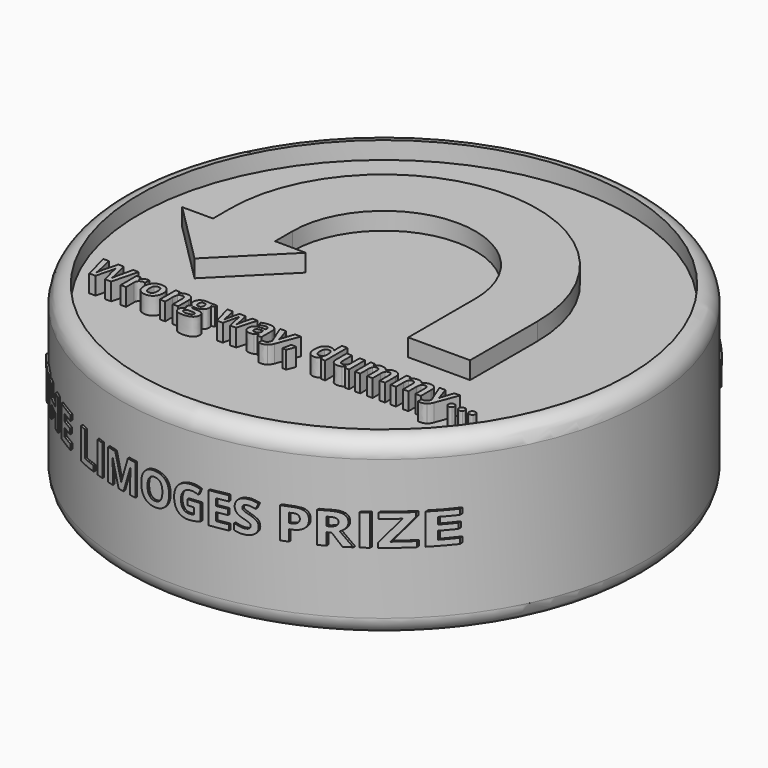
from build123d import *

# Parameters (mm, degrees)
F0_R         = 38.1
F1_DEPTH     = 25.4
F2_R         = 2.54
F3_R         = 35.56
F4_DEPTH     = 2.54
F5_DEPTH     = 2.54
F6_DEPTH     = 2.54
F8_TEXT_SIZE = 6.3120904723
F9_DEPTH     = 15.24
F10_R        = 50.5261755915
F10_R_2      = 38.354
F11_DEPTH    = 25.4
F13_COUNT    = 2
F13_ANGLE    = 180


# Not quite as in the source:
# - Text() gives the source's letters only with a copy of the font that has no kerning and outlines rounded to 1/6400 em; it was checked with that copy


with BuildPart() as f1:
    # F0 (on Top) → F1 (new body)
    with BuildSketch(Plane.XY):
        Circle(F0_R)
    extrude(amount=F1_DEPTH)

    # F2
    f2_edges = [f1.edges().sort_by_distance(p)[0] for p in [
        (-38.1, 0, 25.4),
        (-38.1, 0, 0),
    ]]
    fillet(f2_edges, radius=F2_R)

    # F3 (on face) → F4 (cut)
    with BuildSketch(Plane.XY.offset(25.4)):
        Circle(F3_R)
        with BuildLine():
            Line((-12.6157349895, -15.8383565248), (-11.6065968712, -15.8383565248))
            Line((-11.6065968712, -15.8383565248), (-11.6065968712, -16.2398593857))
            Line((-11.6065968712, -16.2398593857), (-12.0594258709, -16.3557571187))
            add(Edge.make_bspline(
                [(-12.0594258709, -16.3557571187), (-11.9352497284, -16.550299742), (-11.9352497284, -16.7903736176)],
                knots=[0, 0, 0, 1, 1, 1], degree=2))
            add(Edge.make_bspline(
                [(-11.9352497284, -16.7903736176), (-11.9352497284, -17.2564480726), (-12.2601773014, -17.516390131)],
                knots=[0, 0, 0, 1, 1, 1], degree=2))
            add(Edge.make_bspline(
                [(-12.2601773014, -17.516390131), (-12.5851048743, -17.7763321893), (-13.1612821757, -17.7763321893)],
                knots=[0, 0, 0, 1, 1, 1], degree=2))
            Line((-13.1612821757, -17.7763321893), (-13.3036708191, -17.7680537798))
            Line((-13.3036708191, -17.7680537798), (-13.4203963931, -17.7556361656))
            add(Edge.make_bspline(
                [(-13.4203963931, -17.7556361656), (-13.5420890128, -17.848354352), (-13.5420890128, -17.9625964031)],
                knots=[0, 0, 0, 1, 1, 1], degree=2))
            add(Edge.make_bspline(
                [(-13.5420890128, -17.9625964031), (-13.5420890128, -18.1331316389), (-13.1074725139, -18.1331316389)],
                knots=[0, 0, 0, 1, 1, 1], degree=2))
            Line((-13.1074725139, -18.1331316389), (-12.6157349895, -18.1331316389))
            add(Edge.make_bspline(
                [(-12.6157349895, -18.1331316389), (-12.1397264431, -18.1331316389), (-11.8901323966, -18.3376083536)],
                knots=[0, 0, 0, 1, 1, 1], degree=2))
            add(Edge.make_bspline(
                [(-11.8901323966, -18.3376083536), (-11.6405383501, -18.5420850683), (-11.6405383501, -18.9377930425)],
                knots=[0, 0, 0, 1, 1, 1], degree=2))
            add(Edge.make_bspline(
                [(-11.6405383501, -18.9377930425), (-11.6405383501, -19.445259545), (-12.0635650757, -19.7246558657)],
                knots=[0, 0, 0, 1, 1, 1], degree=2))
            add(Edge.make_bspline(
                [(-12.0635650757, -19.7246558657), (-12.4865918013, -20.0040521864), (-13.2780077497, -20.0040521864)],
                knots=[0, 0, 0, 1, 1, 1], degree=2))
            add(Edge.make_bspline(
                [(-13.2780077497, -20.0040521864), (-13.8831594843, -20.0040521864), (-14.2027060911, -19.7929527441)],
                knots=[0, 0, 0, 1, 1, 1], degree=2))
            add(Edge.make_bspline(
                [(-14.2027060911, -19.7929527441), (-14.5222526979, -19.5818533018), (-14.5222526979, -19.2018743057)],
                knots=[0, 0, 0, 1, 1, 1], degree=2))
            add(Edge.make_bspline(
                [(-14.5222526979, -19.2018743057), (-14.5222526979, -18.9402765654), (-14.3591680307, -18.7643603635)],
                knots=[0, 0, 0, 1, 1, 1], degree=2))
            add(Edge.make_bspline(
                [(-14.3591680307, -18.7643603635), (-14.1960833635, -18.5884441615), (-13.8806759615, -18.5131106351)],
                knots=[0, 0, 0, 1, 1, 1], degree=2))
            add(Edge.make_bspline(
                [(-13.8806759615, -18.5131106351), (-14.0023685812, -18.4617844961), (-14.0930171652, -18.3442310812)],
                knots=[0, 0, 0, 1, 1, 1], degree=2))
            add(Edge.make_bspline(
                [(-14.0930171652, -18.3442310812), (-14.1836657493, -18.2266776663), (-14.1836657493, -18.0942231142)],
                knots=[0, 0, 0, 1, 1, 1], degree=2))
            add(Edge.make_bspline(
                [(-14.1836657493, -18.0942231142), (-14.1836657493, -17.9286549242), (-14.0880501195, -17.8189659983)],
                knots=[0, 0, 0, 1, 1, 1], degree=2))
            add(Edge.make_bspline(
                [(-14.0880501195, -17.8189659983), (-13.9924344898, -17.7092770724), (-13.8111373216, -17.6024855898)],
                knots=[0, 0, 0, 1, 1, 1], degree=2))
            add(Edge.make_bspline(
                [(-13.8111373216, -17.6024855898), (-14.038793583, -17.5048003577), (-14.172075976, -17.2874921082)],
                knots=[0, 0, 0, 1, 1, 1], degree=2))
            add(Edge.make_bspline(
                [(-14.172075976, -17.2874921082), (-14.3053583689, -17.0701838588), (-14.3053583689, -16.7746446395)],
                knots=[0, 0, 0, 1, 1, 1], degree=2))
            add(Edge.make_bspline(
                [(-14.3053583689, -16.7746446395), (-14.3053583689, -16.301947457), (-13.9974015355, -16.04324716)],
                knots=[0, 0, 0, 1, 1, 1], degree=2))
            add(Edge.make_bspline(
                [(-13.9974015355, -16.04324716), (-13.689444702, -15.7845468631), (-13.1174066053, -15.7845468631)],
                knots=[0, 0, 0, 1, 1, 1], degree=2))
            add(Edge.make_bspline(
                [(-13.1174066053, -15.7845468631), (-12.9957139857, -15.7845468631), (-12.8289040342, -15.8064846482)],
                knots=[0, 0, 0, 1, 1, 1], degree=2))
            add(Edge.make_bspline(
                [(-12.8289040342, -15.8064846482), (-12.6620940827, -15.8284224334), (-12.6157349895, -15.8383565248)],
                knots=[0, 0, 0, 1, 1, 1], degree=2))
        make_face(mode=Mode.SUBTRACT)
        with BuildLine():
            Line((-1.2834202216, -18.7101367812), (-2.4324634606, -15.8383565248))
            Line((-2.4324634606, -15.8383565248), (-1.5681975085, -15.8383565248))
            Line((-1.5681975085, -15.8383565248), (-1.0226503223, -17.465891833))
            add(Edge.make_bspline(
                [(-1.0226503223, -17.465891833), (-0.9522838415, -17.6778191163), (-0.9266207721, -17.9675634488)],
                knots=[0, 0, 0, 1, 1, 1], degree=2))
            Line((-0.9266207721, -17.9675634488), (-0.910891794, -17.9675634488))
            add(Edge.make_bspline(
                [(-0.910891794, -17.9675634488), (-0.8827452017, -17.7009986629), (-0.7999611067, -17.465891833)],
                knots=[0, 0, 0, 1, 1, 1], degree=2))
            Line((-0.7999611067, -17.465891833), (-0.2643480119, -15.8383565248))
            Line((-0.2643480119, -15.8383565248), (0.5817054393, -15.8383565248))
            Line((0.5817054393, -15.8383565248), (-0.6418434852, -19.1008777097))
            add(Edge.make_bspline(
                [(-0.6418434852, -19.1008777097), (-0.810723039, -19.5537067095), (-1.1224051568, -19.778879448)],
                knots=[0, 0, 0, 1, 1, 1], degree=2))
            add(Edge.make_bspline(
                [(-1.1224051568, -19.778879448), (-1.4340872746, -20.0040521864), (-1.8504912725, -20.0040521864)],
                knots=[0, 0, 0, 1, 1, 1], degree=2))
            add(Edge.make_bspline(
                [(-1.8504912725, -20.0040521864), (-2.0549679873, -20.0040521864), (-2.2511662925, -19.9593487751)],
                knots=[0, 0, 0, 1, 1, 1], degree=2))
            Line((-2.2511662925, -19.9593487751), (-2.2511662925, -19.3335010167))
            add(Edge.make_bspline(
                [(-2.2511662925, -19.3335010167), (-2.108777649, -19.3674424957), (-1.9407259361, -19.3674424957)],
                knots=[0, 0, 0, 1, 1, 1], degree=2))
            add(Edge.make_bspline(
                [(-1.9407259361, -19.3674424957), (-1.7312821757, -19.3674424957), (-1.5748202361, -19.2391271484)],
                knots=[0, 0, 0, 1, 1, 1], degree=2))
            add(Edge.make_bspline(
                [(-1.5748202361, -19.2391271484), (-1.4183582965, -19.1108118011), (-1.3306071558, -18.8525254247)],
                knots=[0, 0, 0, 1, 1, 1], degree=2))
            Line((-1.3306071558, -18.8525254247), (-1.2834202216, -18.7101367812))
        make_face(mode=Mode.SUBTRACT)
        with BuildLine():
            Line((-23.7063201999, -14.9484275033), (-24.669099225, -18.730832805))
            Line((-24.669099225, -18.730832805), (-25.5822077931, -18.730832805))
            Line((-25.5822077931, -18.730832805), (-26.0946413413, -16.7440145244))
            add(Edge.make_bspline(
                [(-26.0946413413, -16.7440145244), (-26.1227879337, -16.6380508828), (-26.1914987325, -16.3056727412)],
                knots=[0, 0, 0, 1, 1, 1], degree=2))
            add(Edge.make_bspline(
                [(-26.1914987325, -16.3056727412), (-26.2602095314, -15.9732945997), (-26.2701436228, -15.8590525486)],
                knots=[0, 0, 0, 1, 1, 1], degree=2))
            add(Edge.make_bspline(
                [(-26.2701436228, -15.8590525486), (-26.2858726009, -15.9989576692), (-26.3479606721, -16.3081562641)],
                knots=[0, 0, 0, 1, 1, 1], degree=2))
            add(Edge.make_bspline(
                [(-26.3479606721, -16.3081562641), (-26.4100487434, -16.617354859), (-26.4439902224, -16.7489815701)],
                knots=[0, 0, 0, 1, 1, 1], degree=2))
            Line((-26.4439902224, -16.7489815701), (-26.9531124068, -18.730832805))
            Line((-26.9531124068, -18.730832805), (-27.863737452, -18.730832805))
            Line((-27.863737452, -18.730832805), (-28.829, -14.9484275033))
            Line((-28.829, -14.9484275033), (-28.0400675744, -14.9484275033))
            Line((-28.0400675744, -14.9484275033), (-27.5557806185, -17.0130628332))
            add(Edge.make_bspline(
                [(-27.5557806185, -17.0130628332), (-27.4291209531, -17.5851009298), (-27.3728277685, -18.0039884507)],
                knots=[0, 0, 0, 1, 1, 1], degree=2))
            add(Edge.make_bspline(
                [(-27.3728277685, -18.0039884507), (-27.3570987905, -17.8566327615), (-27.3012195263, -17.5474341666)],
                knots=[0, 0, 0, 1, 1, 1], degree=2))
            add(Edge.make_bspline(
                [(-27.3012195263, -17.5474341666), (-27.2453402622, -17.2382355717), (-27.1964976461, -17.0677003359)],
                knots=[0, 0, 0, 1, 1, 1], degree=2))
            Line((-27.1964976461, -17.0677003359), (-26.6451555733, -14.9484275033))
            Line((-26.6451555733, -14.9484275033), (-25.8876811038, -14.9484275033))
            Line((-25.8876811038, -14.9484275033), (-25.3363390309, -17.0677003359))
            add(Edge.make_bspline(
                [(-25.3363390309, -17.0677003359), (-25.2999140291, -17.2092611384), (-25.2456904469, -17.5019029143)],
                knots=[0, 0, 0, 1, 1, 1], degree=2))
            add(Edge.make_bspline(
                [(-25.2456904469, -17.5019029143), (-25.1914668646, -17.7945446902), (-25.1633202723, -18.0039884507)],
                knots=[0, 0, 0, 1, 1, 1], degree=2))
            add(Edge.make_bspline(
                [(-25.1633202723, -18.0039884507), (-25.1376572029, -17.8019952588), (-25.0805361773, -17.5006611529)],
                knots=[0, 0, 0, 1, 1, 1], degree=2))
            add(Edge.make_bspline(
                [(-25.0805361773, -17.5006611529), (-25.0234151517, -17.199327047), (-24.9770560585, -17.0130628332)],
                knots=[0, 0, 0, 1, 1, 1], degree=2))
            Line((-24.9770560585, -17.0130628332), (-24.4960804664, -14.9484275033))
            Line((-24.4960804664, -14.9484275033), (-23.7063201999, -14.9484275033))
        make_face(mode=Mode.SUBTRACT)
        with BuildLine():
            add(Edge.make_bspline(
                [(-22.1760562034, -15.9331443136), (-21.9471581806, -15.7845468631), (-21.6781098718, -15.7845468631)],
                knots=[0, 0, 0, 1, 1, 1], degree=2))
            add(Edge.make_bspline(
                [(-21.6781098718, -15.7845468631), (-21.5175087275, -15.7845468631), (-21.4115450858, -15.8077264097)],
                knots=[0, 0, 0, 1, 1, 1], degree=2))
            Line((-21.4115450858, -15.8077264097), (-21.4711496342, -16.5469883782))
            add(Edge.make_bspline(
                [(-21.4711496342, -16.5469883782), (-21.5671791845, -16.5213253088), (-21.7037729413, -16.5213253088)],
                knots=[0, 0, 0, 1, 1, 1], degree=2))
            add(Edge.make_bspline(
                [(-21.7037729413, -16.5213253088), (-22.0812684146, -16.5213253088), (-22.2923678569, -16.7154540116)],
                knots=[0, 0, 0, 1, 1, 1], degree=2))
            add(Edge.make_bspline(
                [(-22.2923678569, -16.7154540116), (-22.5034672992, -16.9095827144), (-22.5034672992, -17.2589315954)],
                knots=[0, 0, 0, 1, 1, 1], degree=2))
            Line((-22.5034672992, -17.2589315954), (-22.5034672992, -18.730832805))
            Line((-22.5034672992, -18.730832805), (-23.2923997248, -18.730832805))
            Line((-23.2923997248, -18.730832805), (-23.2923997248, -15.8383565248))
            Line((-23.2923997248, -15.8383565248), (-22.6946985587, -15.8383565248))
            Line((-22.6946985587, -15.8383565248), (-22.5779729847, -16.3251270036))
            Line((-22.5779729847, -16.3251270036), (-22.539892301, -16.3251270036))
            add(Edge.make_bspline(
                [(-22.539892301, -16.3251270036), (-22.4049542261, -16.0817417642), (-22.1760562034, -15.9331443136)],
                knots=[0, 0, 0, 1, 1, 1], degree=2))
        make_face(mode=Mode.SUBTRACT)
        with BuildLine():
            add(Edge.make_bspline(
                [(-18.4288341421, -16.4853142274), (-18.2582989064, -16.8243150966), (-18.2582989064, -17.2796276192)],
                knots=[0, 0, 0, 1, 1, 1], degree=2))
            add(Edge.make_bspline(
                [(-18.2582989064, -17.2796276192), (-18.2582989064, -17.9857759498), (-18.630827334, -18.3843813673)],
                knots=[0, 0, 0, 1, 1, 1], degree=2))
            add(Edge.make_bspline(
                [(-18.630827334, -18.3843813673), (-19.0033557616, -18.7829867848), (-19.6681120446, -18.7829867848)],
                knots=[0, 0, 0, 1, 1, 1], degree=2))
            add(Edge.make_bspline(
                [(-19.6681120446, -18.7829867848), (-20.0845160426, -18.7829867848), (-20.402820888, -18.6004478553)],
                knots=[0, 0, 0, 1, 1, 1], degree=2))
            add(Edge.make_bspline(
                [(-20.402820888, -18.6004478553), (-20.7211257333, -18.4179089258), (-20.8916609691, -18.0764245338)],
                knots=[0, 0, 0, 1, 1, 1], degree=2))
            add(Edge.make_bspline(
                [(-20.8916609691, -18.0764245338), (-21.0621962048, -17.7349401418), (-21.0621962048, -17.2796276192)],
                knots=[0, 0, 0, 1, 1, 1], degree=2))
            add(Edge.make_bspline(
                [(-21.0621962048, -17.2796276192), (-21.0621962048, -16.5709957658), (-20.6925652205, -16.1777713144)],
                knots=[0, 0, 0, 1, 1, 1], degree=2))
            add(Edge.make_bspline(
                [(-20.6925652205, -16.1777713144), (-20.3229342363, -15.7845468631), (-19.6523830666, -15.7845468631)],
                knots=[0, 0, 0, 1, 1, 1], degree=2))
            add(Edge.make_bspline(
                [(-19.6523830666, -15.7845468631), (-19.2359790686, -15.7845468631), (-18.9176742232, -15.9654301107)],
                knots=[0, 0, 0, 1, 1, 1], degree=2))
            add(Edge.make_bspline(
                [(-18.9176742232, -15.9654301107), (-18.5993693779, -16.1463133583), (-18.4288341421, -16.4853142274)],
                knots=[0, 0, 0, 1, 1, 1], degree=2))
        make_face(mode=Mode.SUBTRACT)
        with BuildLine():
            Line((-14.936173173, -16.8450111203), (-14.936173173, -18.730832805))
            Line((-14.936173173, -18.730832805), (-15.7251055986, -18.730832805))
            Line((-15.7251055986, -18.730832805), (-15.7251055986, -17.0412094255))
            add(Edge.make_bspline(
                [(-15.7251055986, -17.0412094255), (-15.7251055986, -16.7282855463), (-15.8364502064, -16.5718236067)],
                knots=[0, 0, 0, 1, 1, 1], degree=2))
            add(Edge.make_bspline(
                [(-15.8364502064, -16.5718236067), (-15.9477948142, -16.4153616671), (-16.1911800536, -16.4153616671)],
                knots=[0, 0, 0, 1, 1, 1], degree=2))
            add(Edge.make_bspline(
                [(-16.1911800536, -16.4153616671), (-16.5223164337, -16.4153616671), (-16.6696721228, -16.6363952009)],
                knots=[0, 0, 0, 1, 1, 1], degree=2))
            add(Edge.make_bspline(
                [(-16.6696721228, -16.6363952009), (-16.817027812, -16.8574287346), (-16.817027812, -17.3698622828)],
                knots=[0, 0, 0, 1, 1, 1], degree=2))
            Line((-16.817027812, -17.3698622828), (-16.817027812, -18.730832805))
            Line((-16.817027812, -18.730832805), (-17.6059602376, -18.730832805))
            Line((-17.6059602376, -18.730832805), (-17.6059602376, -15.8383565248))
            Line((-17.6059602376, -15.8383565248), (-17.0032920258, -15.8383565248))
            Line((-17.0032920258, -15.8383565248), (-16.8973283842, -16.2084014296))
            Line((-16.8973283842, -16.2084014296), (-16.8534528138, -16.2084014296))
            add(Edge.make_bspline(
                [(-16.8534528138, -16.2084014296), (-16.7209982618, -15.9989576692), (-16.4896167162, -15.8917522661)],
                knots=[0, 0, 0, 1, 1, 1], degree=2))
            add(Edge.make_bspline(
                [(-16.4896167162, -15.8917522661), (-16.2582351706, -15.7845468631), (-15.9635237923, -15.7845468631)],
                knots=[0, 0, 0, 1, 1, 1], degree=2))
            add(Edge.make_bspline(
                [(-15.9635237923, -15.7845468631), (-15.4585408126, -15.7845468631), (-15.1973569928, -16.0573204562)],
                knots=[0, 0, 0, 1, 1, 1], degree=2))
            add(Edge.make_bspline(
                [(-15.1973569928, -16.0573204562), (-14.936173173, -16.3300940493), (-14.936173173, -16.8450111203)],
                knots=[0, 0, 0, 1, 1, 1], degree=2))
        make_face(mode=Mode.SUBTRACT)
        with BuildLine():
            Line((-6.51785855, -18.730832805), (-7.3763296154, -18.730832805))
            Line((-7.3763296154, -18.730832805), (-7.599018831, -17.7192111638))
            Line((-7.599018831, -17.7192111638), (-7.898697255, -16.4410247366))
            Line((-7.898697255, -16.4410247366), (-7.9169097559, -16.4410247366))
            Line((-7.9169097559, -16.4410247366), (-8.4450722822, -18.730832805))
            Line((-8.4450722822, -18.730832805), (-9.2936092562, -18.730832805))
            Line((-9.2936092562, -18.730832805), (-10.1156553198, -15.8383565248))
            Line((-10.1156553198, -15.8383565248), (-9.329206417, -15.8383565248))
            Line((-9.329206417, -15.8383565248), (-8.9955865141, -17.1190264748))
            add(Edge.make_bspline(
                [(-8.9955865141, -17.1190264748), (-8.9152859419, -17.4634083102), (-8.8325018469, -18.0685600448)],
                knots=[0, 0, 0, 1, 1, 1], degree=2))
            Line((-8.8325018469, -18.0685600448), (-8.8176007098, -18.0685600448))
            add(Edge.make_bspline(
                [(-8.8176007098, -18.0685600448), (-8.8068387774, -17.8715338986), (-8.7265382053, -17.4451958092)],
                knots=[0, 0, 0, 1, 1, 1], degree=2))
            Line((-8.7265382053, -17.4451958092), (-8.6851461577, -17.2249901165))
            Line((-8.6851461577, -17.2249901165), (-8.3283467082, -15.8383565248))
            Line((-8.3283467082, -15.8383565248), (-7.4591137104, -15.8383565248))
            Line((-7.4591137104, -15.8383565248), (-7.1205267618, -17.2249901165))
            add(Edge.make_bspline(
                [(-7.1205267618, -17.2249901165), (-7.1097648294, -17.282111142), (-7.0878270443, -17.3934557499)],
                knots=[0, 0, 0, 1, 1, 1], degree=2))
            add(Edge.make_bspline(
                [(-7.0878270443, -17.3934557499), (-7.0658892591, -17.5048003577), (-7.0451932353, -17.6302182616)],
                knots=[0, 0, 0, 1, 1, 1], degree=2))
            add(Edge.make_bspline(
                [(-7.0451932353, -17.6302182616), (-7.0244972116, -17.7556361656), (-7.0075264721, -17.8756731034)],
                knots=[0, 0, 0, 1, 1, 1], degree=2))
            add(Edge.make_bspline(
                [(-7.0075264721, -17.8756731034), (-6.9905557326, -17.9957100412), (-6.9880722097, -18.0685600448)],
                knots=[0, 0, 0, 1, 1, 1], degree=2))
            Line((-6.9880722097, -18.0685600448), (-6.9731710726, -18.0685600448))
            add(Edge.make_bspline(
                [(-6.9731710726, -18.0685600448), (-6.9491636851, -17.882295831), (-6.8899730571, -17.5577821785)],
                knots=[0, 0, 0, 1, 1, 1], degree=2))
            add(Edge.make_bspline(
                [(-6.8899730571, -17.5577821785), (-6.8307824292, -17.233268526), (-6.8042915188, -17.1190264748)],
                knots=[0, 0, 0, 1, 1, 1], degree=2))
            Line((-6.8042915188, -17.1190264748), (-6.4582540016, -15.8383565248))
            Line((-6.4582540016, -15.8383565248), (-5.6842227131, -15.8383565248))
            Line((-5.6842227131, -15.8383565248), (-6.51785855, -18.730832805))
        make_face(mode=Mode.SUBTRACT)
        with BuildLine():
            Line((-2.8314827986, -18.730832805), (-3.3819970305, -18.730832805))
            Line((-3.3819970305, -18.730832805), (-3.5351476063, -18.3376083536))
            Line((-3.5351476063, -18.3376083536), (-3.55584363, -18.3376083536))
            add(Edge.make_bspline(
                [(-3.55584363, -18.3376083536), (-3.7545254581, -18.5884441615), (-3.9656249004, -18.6857154732)],
                knots=[0, 0, 0, 1, 1, 1], degree=2))
            add(Edge.make_bspline(
                [(-3.9656249004, -18.6857154732), (-4.1767243427, -18.7829867848), (-4.5153112914, -18.7829867848)],
                knots=[0, 0, 0, 1, 1, 1], degree=2))
            add(Edge.make_bspline(
                [(-4.5153112914, -18.7829867848), (-4.9317152893, -18.7829867848), (-5.170961324, -18.5445685912)],
                knots=[0, 0, 0, 1, 1, 1], degree=2))
            add(Edge.make_bspline(
                [(-5.170961324, -18.5445685912), (-5.4102073586, -18.3061503975), (-5.4102073586, -17.8665668529)],
                knots=[0, 0, 0, 1, 1, 1], degree=2))
            add(Edge.make_bspline(
                [(-5.4102073586, -17.8665668529), (-5.4102073586, -17.4062872846), (-5.0881772289, -17.1877372737)],
                knots=[0, 0, 0, 1, 1, 1], degree=2))
            add(Edge.make_bspline(
                [(-5.0881772289, -17.1877372737), (-4.7661470993, -16.9691872629), (-4.1171197943, -16.9460077162)],
                knots=[0, 0, 0, 1, 1, 1], degree=2))
            Line((-4.1171197943, -16.9460077162), (-3.6146203375, -16.9302787382))
            Line((-3.6146203375, -16.9302787382), (-3.6146203375, -16.8036190728))
            add(Edge.make_bspline(
                [(-3.6146203375, -16.8036190728), (-3.6146203375, -16.3640355282), (-4.0649658144, -16.3640355282)],
                knots=[0, 0, 0, 1, 1, 1], degree=2))
            add(Edge.make_bspline(
                [(-4.0649658144, -16.3640355282), (-4.4118311726, -16.3640355282), (-4.8803891504, -16.5734792886)],
                knots=[0, 0, 0, 1, 1, 1], degree=2))
            Line((-4.8803891504, -16.5734792886), (-5.1411590498, -16.0403497167))
            add(Edge.make_bspline(
                [(-5.1411590498, -16.0403497167), (-4.6419709568, -15.7787519764), (-4.0343356993, -15.7787519764)],
                knots=[0, 0, 0, 1, 1, 1], degree=2))
            add(Edge.make_bspline(
                [(-4.0343356993, -15.7787519764), (-3.4523635113, -15.7787519764), (-3.1419231549, -16.0324852277)],
                knots=[0, 0, 0, 1, 1, 1], degree=2))
            add(Edge.make_bspline(
                [(-3.1419231549, -16.0324852277), (-2.8314827986, -16.2862184789), (-2.8314827986, -16.8036190728)],
                knots=[0, 0, 0, 1, 1, 1], degree=2))
            Line((-2.8314827986, -16.8036190728), (-2.8314827986, -18.730832805))
        make_face(mode=Mode.SUBTRACT)
        with BuildLine():
            Line((1.7307486782, -18.114919138), (1.7688293619, -18.1745236864))
            add(Edge.make_bspline(
                [(1.7688293619, -18.1745236864), (1.634719128, -18.696891326), (1.3135168393, -19.4138015889)],
                knots=[0, 0, 0, 1, 1, 1], degree=2))
            Line((1.3135168393, -19.4138015889), (0.7447901065, -19.4138015889))
            add(Edge.make_bspline(
                [(0.7447901065, -19.4138015889), (0.9128418194, -18.7258657593), (1.0063878467, -18.114919138)],
                knots=[0, 0, 0, 1, 1, 1], degree=2))
            Line((1.0063878467, -18.114919138), (1.7307486782, -18.114919138))
        make_face(mode=Mode.SUBTRACT)
        with BuildLine():
            Line((21.88288093, -18.7101367812), (20.733837691, -15.8383565248))
            Line((20.733837691, -15.8383565248), (21.5981036431, -15.8383565248))
            Line((21.5981036431, -15.8383565248), (22.1436508293, -17.465891833))
            add(Edge.make_bspline(
                [(22.1436508293, -17.465891833), (22.2140173101, -17.6778191163), (22.2396803795, -17.9675634488)],
                knots=[0, 0, 0, 1, 1, 1], degree=2))
            Line((22.2396803795, -17.9675634488), (22.2554093576, -17.9675634488))
            add(Edge.make_bspline(
                [(22.2554093576, -17.9675634488), (22.2835559499, -17.7009986629), (22.3663400449, -17.465891833)],
                knots=[0, 0, 0, 1, 1, 1], degree=2))
            Line((22.3663400449, -17.465891833), (22.9019531397, -15.8383565248))
            Line((22.9019531397, -15.8383565248), (23.7480065909, -15.8383565248))
            Line((23.7480065909, -15.8383565248), (22.5244576664, -19.1008777097))
            add(Edge.make_bspline(
                [(22.5244576664, -19.1008777097), (22.3555781126, -19.5537067095), (22.0438959948, -19.778879448)],
                knots=[0, 0, 0, 1, 1, 1], degree=2))
            add(Edge.make_bspline(
                [(22.0438959948, -19.778879448), (21.732213877, -20.0040521864), (21.315809879, -20.0040521864)],
                knots=[0, 0, 0, 1, 1, 1], degree=2))
            add(Edge.make_bspline(
                [(21.315809879, -20.0040521864), (21.1113331643, -20.0040521864), (20.9151348591, -19.9593487751)],
                knots=[0, 0, 0, 1, 1, 1], degree=2))
            Line((20.9151348591, -19.9593487751), (20.9151348591, -19.3335010167))
            add(Edge.make_bspline(
                [(20.9151348591, -19.3335010167), (21.0575235026, -19.3674424957), (21.2255752155, -19.3674424957)],
                knots=[0, 0, 0, 1, 1, 1], degree=2))
            add(Edge.make_bspline(
                [(21.2255752155, -19.3674424957), (21.4350189759, -19.3674424957), (21.5914809155, -19.2391271484)],
                knots=[0, 0, 0, 1, 1, 1], degree=2))
            add(Edge.make_bspline(
                [(21.5914809155, -19.2391271484), (21.7479428551, -19.1108118011), (21.8356939958, -18.8525254247)],
                knots=[0, 0, 0, 1, 1, 1], degree=2))
            Line((21.8356939958, -18.8525254247), (21.88288093, -18.7101367812))
        make_face(mode=Mode.SUBTRACT)
        with BuildLine():
            add(Edge.make_bspline(
                [(24.169791555, -18.6853015527), (24.0509963786, -18.5702316606), (24.0509963786, -18.3607879002)],
                knots=[0, 0, 0, 1, 1, 1], degree=2))
            add(Edge.make_bspline(
                [(24.0509963786, -18.3607879002), (24.0509963786, -18.1438935712), (24.1673080322, -18.0325489634)],
                knots=[0, 0, 0, 1, 1, 1], degree=2))
            add(Edge.make_bspline(
                [(24.1673080322, -18.0325489634), (24.2836196857, -17.9212043556), (24.5063089013, -17.9212043556)],
                knots=[0, 0, 0, 1, 1, 1], degree=2))
            add(Edge.make_bspline(
                [(24.5063089013, -17.9212043556), (24.7207197074, -17.9212043556), (24.8382731223, -18.0350324863)],
                knots=[0, 0, 0, 1, 1, 1], degree=2))
            add(Edge.make_bspline(
                [(24.8382731223, -18.0350324863), (24.9558265373, -18.148860617), (24.9558265373, -18.3607879002)],
                knots=[0, 0, 0, 1, 1, 1], degree=2))
            add(Edge.make_bspline(
                [(24.9558265373, -18.3607879002), (24.9558265373, -18.5652646149), (24.8370313609, -18.6828180299)],
                knots=[0, 0, 0, 1, 1, 1], degree=2))
            add(Edge.make_bspline(
                [(24.8370313609, -18.6828180299), (24.7182361845, -18.8003714448), (24.5063089013, -18.8003714448)],
                knots=[0, 0, 0, 1, 1, 1], degree=2))
            add(Edge.make_bspline(
                [(24.5063089013, -18.8003714448), (24.2885867314, -18.8003714448), (24.169791555, -18.6853015527)],
                knots=[0, 0, 0, 1, 1, 1], degree=2))
        make_face(mode=Mode.SUBTRACT)
        with BuildLine():
            add(Edge.make_bspline(
                [(25.6806012892, -18.6853015527), (25.5618061128, -18.5702316606), (25.5618061128, -18.3607879002)],
                knots=[0, 0, 0, 1, 1, 1], degree=2))
            add(Edge.make_bspline(
                [(25.5618061128, -18.3607879002), (25.5618061128, -18.1438935712), (25.6781177664, -18.0325489634)],
                knots=[0, 0, 0, 1, 1, 1], degree=2))
            add(Edge.make_bspline(
                [(25.6781177664, -18.0325489634), (25.7944294199, -17.9212043556), (26.0171186355, -17.9212043556)],
                knots=[0, 0, 0, 1, 1, 1], degree=2))
            add(Edge.make_bspline(
                [(26.0171186355, -17.9212043556), (26.2315294416, -17.9212043556), (26.3490828565, -18.0350324863)],
                knots=[0, 0, 0, 1, 1, 1], degree=2))
            add(Edge.make_bspline(
                [(26.3490828565, -18.0350324863), (26.4666362715, -18.148860617), (26.4666362715, -18.3607879002)],
                knots=[0, 0, 0, 1, 1, 1], degree=2))
            add(Edge.make_bspline(
                [(26.4666362715, -18.3607879002), (26.4666362715, -18.5652646149), (26.3478410951, -18.6828180299)],
                knots=[0, 0, 0, 1, 1, 1], degree=2))
            add(Edge.make_bspline(
                [(26.3478410951, -18.6828180299), (26.2290459187, -18.8003714448), (26.0171186355, -18.8003714448)],
                knots=[0, 0, 0, 1, 1, 1], degree=2))
            add(Edge.make_bspline(
                [(26.0171186355, -18.8003714448), (25.7993964656, -18.8003714448), (25.6806012892, -18.6853015527)],
                knots=[0, 0, 0, 1, 1, 1], degree=2))
        make_face(mode=Mode.SUBTRACT)
        with BuildLine():
            add(Edge.make_bspline(
                [(27.1914110234, -18.6853015527), (27.072615847, -18.5702316606), (27.072615847, -18.3607879002)],
                knots=[0, 0, 0, 1, 1, 1], degree=2))
            add(Edge.make_bspline(
                [(27.072615847, -18.3607879002), (27.072615847, -18.1438935712), (27.1889275005, -18.0325489634)],
                knots=[0, 0, 0, 1, 1, 1], degree=2))
            add(Edge.make_bspline(
                [(27.1889275005, -18.0325489634), (27.3052391541, -17.9212043556), (27.5279283697, -17.9212043556)],
                knots=[0, 0, 0, 1, 1, 1], degree=2))
            add(Edge.make_bspline(
                [(27.5279283697, -17.9212043556), (27.7423391758, -17.9212043556), (27.8598925907, -18.0350324863)],
                knots=[0, 0, 0, 1, 1, 1], degree=2))
            add(Edge.make_bspline(
                [(27.8598925907, -18.0350324863), (27.9774460056, -18.148860617), (27.9774460056, -18.3607879002)],
                knots=[0, 0, 0, 1, 1, 1], degree=2))
            add(Edge.make_bspline(
                [(27.9774460056, -18.3607879002), (27.9774460056, -18.5652646149), (27.8586508293, -18.6828180299)],
                knots=[0, 0, 0, 1, 1, 1], degree=2))
            add(Edge.make_bspline(
                [(27.8586508293, -18.6828180299), (27.7398556529, -18.8003714448), (27.5279283697, -18.8003714448)],
                knots=[0, 0, 0, 1, 1, 1], degree=2))
            add(Edge.make_bspline(
                [(27.5279283697, -18.8003714448), (27.3102061998, -18.8003714448), (27.1914110234, -18.6853015527)],
                knots=[0, 0, 0, 1, 1, 1], degree=2))
        make_face(mode=Mode.SUBTRACT)
        with BuildLine():
            add(Edge.make_bspline(
                [(5.644780691, -18.3558208545), (5.3757323821, -18.7829867848), (4.8243903093, -18.7829867848)],
                knots=[0, 0, 0, 1, 1, 1], degree=2))
            add(Edge.make_bspline(
                [(4.8243903093, -18.7829867848), (4.3152681249, -18.7829867848), (4.0242820309, -18.3868648901)],
                knots=[0, 0, 0, 1, 1, 1], degree=2))
            add(Edge.make_bspline(
                [(4.0242820309, -18.3868648901), (3.7332959368, -17.9907429955), (3.7332959368, -17.2895617106)],
                knots=[0, 0, 0, 1, 1, 1], degree=2))
            add(Edge.make_bspline(
                [(3.7332959368, -17.2895617106), (3.7332959368, -16.5784463343), (4.0292490766, -16.1814965987)],
                knots=[0, 0, 0, 1, 1, 1], degree=2))
            add(Edge.make_bspline(
                [(4.0292490766, -16.1814965987), (4.3252022163, -15.7845468631), (4.845086333, -15.7845468631)],
                knots=[0, 0, 0, 1, 1, 1], degree=2))
            add(Edge.make_bspline(
                [(4.845086333, -15.7845468631), (5.3914613602, -15.7845468631), (5.6787221699, -16.2084014296)],
                knots=[0, 0, 0, 1, 1, 1], degree=2))
            Line((5.6787221699, -16.2084014296), (5.7043852394, -16.2084014296))
            add(Edge.make_bspline(
                [(5.7043852394, -16.2084014296), (5.644780691, -15.884715618), (5.644780691, -15.6313962873)],
                knots=[0, 0, 0, 1, 1, 1], degree=2))
            Line((5.644780691, -15.6313962873), (5.644780691, -14.7050422639))
            Line((5.644780691, -14.7050422639), (6.4361966394, -14.7050422639))
            Line((6.4361966394, -14.7050422639), (6.4361966394, -18.730832805))
            Line((6.4361966394, -18.730832805), (5.8310449048, -18.730832805))
            Line((5.8310449048, -18.730832805), (5.6787221699, -18.3558208545))
            Line((5.6787221699, -18.3558208545), (5.644780691, -18.3558208545))
        make_face(mode=Mode.SUBTRACT)
        with BuildLine():
            Line((9.9156121533, -18.730832805), (9.3104604186, -18.730832805))
            Line((9.3104604186, -18.730832805), (9.204496777, -18.3607879002))
            Line((9.204496777, -18.3607879002), (9.1631047295, -18.3607879002))
            add(Edge.make_bspline(
                [(9.1631047295, -18.3607879002), (9.0364450641, -18.5627810921), (8.8034078366, -18.6728839385)],
                knots=[0, 0, 0, 1, 1, 1], degree=2))
            add(Edge.make_bspline(
                [(8.8034078366, -18.6728839385), (8.5703706091, -18.7829867848), (8.273175708, -18.7829867848)],
                knots=[0, 0, 0, 1, 1, 1], degree=2))
            add(Edge.make_bspline(
                [(8.273175708, -18.7829867848), (7.7632256826, -18.7829867848), (7.5045253857, -18.5097992713)],
                knots=[0, 0, 0, 1, 1, 1], degree=2))
            add(Edge.make_bspline(
                [(7.5045253857, -18.5097992713), (7.2458250887, -18.2366117577), (7.2458250887, -17.7241782095)],
                knots=[0, 0, 0, 1, 1, 1], degree=2))
            Line((7.2458250887, -17.7241782095), (7.2458250887, -15.8383565248))
            Line((7.2458250887, -15.8383565248), (8.0347575143, -15.8383565248))
            Line((8.0347575143, -15.8383565248), (8.0347575143, -17.5279799043))
            add(Edge.make_bspline(
                [(8.0347575143, -17.5279799043), (8.0347575143, -17.8409037835), (8.1461021221, -17.9973657231)],
                knots=[0, 0, 0, 1, 1, 1], degree=2))
            add(Edge.make_bspline(
                [(8.1461021221, -17.9973657231), (8.2574467299, -18.1538276627), (8.5008319693, -18.1538276627)],
                knots=[0, 0, 0, 1, 1, 1], degree=2))
            add(Edge.make_bspline(
                [(8.5008319693, -18.1538276627), (8.8319683494, -18.1538276627), (8.9793240385, -17.9327941289)],
                knots=[0, 0, 0, 1, 1, 1], degree=2))
            add(Edge.make_bspline(
                [(8.9793240385, -17.9327941289), (9.1266797277, -17.7117605952), (9.1266797277, -17.199327047)],
                knots=[0, 0, 0, 1, 1, 1], degree=2))
            Line((9.1266797277, -17.199327047), (9.1266797277, -15.8383565248))
            Line((9.1266797277, -15.8383565248), (9.9156121533, -15.8383565248))
            Line((9.9156121533, -15.8383565248), (9.9156121533, -18.730832805))
        make_face(mode=Mode.SUBTRACT)
        with BuildLine():
            Line((13.3329395959, -17.2796276192), (13.3329395959, -18.730832805))
            Line((13.3329395959, -18.730832805), (12.5440071703, -18.730832805))
            Line((12.5440071703, -18.730832805), (12.5440071703, -17.0412094255))
            add(Edge.make_bspline(
                [(12.5440071703, -17.0412094255), (12.5440071703, -16.7282855463), (12.4392852901, -16.5718236067)],
                knots=[0, 0, 0, 1, 1, 1], degree=2))
            add(Edge.make_bspline(
                [(12.4392852901, -16.5718236067), (12.3345634099, -16.4153616671), (12.1093906714, -16.4153616671)],
                knots=[0, 0, 0, 1, 1, 1], degree=2))
            add(Edge.make_bspline(
                [(12.1093906714, -16.4153616671), (11.8064008836, -16.4153616671), (11.6693932063, -16.6380508828)],
                knots=[0, 0, 0, 1, 1, 1], degree=2))
            add(Edge.make_bspline(
                [(11.6693932063, -16.6380508828), (11.5323855291, -16.8607400984), (11.5323855291, -17.3698622828)],
                knots=[0, 0, 0, 1, 1, 1], degree=2))
            Line((11.5323855291, -17.3698622828), (11.5323855291, -18.730832805))
            Line((11.5323855291, -18.730832805), (10.7434531035, -18.730832805))
            Line((10.7434531035, -18.730832805), (10.7434531035, -15.8383565248))
            Line((10.7434531035, -15.8383565248), (11.3461213153, -15.8383565248))
            Line((11.3461213153, -15.8383565248), (11.4520849569, -16.2084014296))
            Line((11.4520849569, -16.2084014296), (11.4959605273, -16.2084014296))
            add(Edge.make_bspline(
                [(11.4959605273, -16.2084014296), (11.6126861013, -16.0088917606), (11.8324778735, -15.8967193118)],
                knots=[0, 0, 0, 1, 1, 1], degree=2))
            add(Edge.make_bspline(
                [(11.8324778735, -15.8967193118), (12.0522696458, -15.7845468631), (12.3370469327, -15.7845468631)],
                knots=[0, 0, 0, 1, 1, 1], degree=2))
            add(Edge.make_bspline(
                [(12.3370469327, -15.7845468631), (12.9860742377, -15.7845468631), (13.2170418628, -16.2084014296)],
                knots=[0, 0, 0, 1, 1, 1], degree=2))
            Line((13.2170418628, -16.2084014296), (13.2865805026, -16.2084014296))
            add(Edge.make_bspline(
                [(13.2865805026, -16.2084014296), (13.4033060766, -16.0064082377), (13.629306656, -15.8954775504)],
                knots=[0, 0, 0, 1, 1, 1], degree=2))
            add(Edge.make_bspline(
                [(13.629306656, -15.8954775504), (13.8553072355, -15.7845468631), (14.1400845223, -15.7845468631)],
                knots=[0, 0, 0, 1, 1, 1], degree=2))
            add(Edge.make_bspline(
                [(14.1400845223, -15.7845468631), (14.6318220468, -15.7845468631), (14.8838996161, -16.0366244324)],
                knots=[0, 0, 0, 1, 1, 1], degree=2))
            add(Edge.make_bspline(
                [(14.8838996161, -16.0366244324), (15.1359771855, -16.2887020018), (15.1359771855, -16.8450111203)],
                knots=[0, 0, 0, 1, 1, 1], degree=2))
            Line((15.1359771855, -16.8450111203), (15.1359771855, -18.730832805))
            Line((15.1359771855, -18.730832805), (14.3445612371, -18.730832805))
            Line((14.3445612371, -18.730832805), (14.3445612371, -17.0412094255))
            add(Edge.make_bspline(
                [(14.3445612371, -17.0412094255), (14.3445612371, -16.7282855463), (14.2398393568, -16.5718236067)],
                knots=[0, 0, 0, 1, 1, 1], degree=2))
            add(Edge.make_bspline(
                [(14.2398393568, -16.5718236067), (14.1351174766, -16.4153616671), (13.9099447382, -16.4153616671)],
                knots=[0, 0, 0, 1, 1, 1], degree=2))
            add(Edge.make_bspline(
                [(13.9099447382, -16.4153616671), (13.6202004056, -16.4153616671), (13.4765700007, -16.6223219047)],
                knots=[0, 0, 0, 1, 1, 1], degree=2))
            add(Edge.make_bspline(
                [(13.4765700007, -16.6223219047), (13.3329395959, -16.8292821423), (13.3329395959, -17.2796276192)],
                knots=[0, 0, 0, 1, 1, 1], degree=2))
        make_face(mode=Mode.SUBTRACT)
        with BuildLine():
            Line((18.5350921272, -17.2796276192), (18.5350921272, -18.730832805))
            Line((18.5350921272, -18.730832805), (17.7461597016, -18.730832805))
            Line((17.7461597016, -18.730832805), (17.7461597016, -17.0412094255))
            add(Edge.make_bspline(
                [(17.7461597016, -17.0412094255), (17.7461597016, -16.7282855463), (17.6414378214, -16.5718236067)],
                knots=[0, 0, 0, 1, 1, 1], degree=2))
            add(Edge.make_bspline(
                [(17.6414378214, -16.5718236067), (17.5367159412, -16.4153616671), (17.3115432027, -16.4153616671)],
                knots=[0, 0, 0, 1, 1, 1], degree=2))
            add(Edge.make_bspline(
                [(17.3115432027, -16.4153616671), (17.0085534149, -16.4153616671), (16.8715457377, -16.6380508828)],
                knots=[0, 0, 0, 1, 1, 1], degree=2))
            add(Edge.make_bspline(
                [(16.8715457377, -16.6380508828), (16.7345380604, -16.8607400984), (16.7345380604, -17.3698622828)],
                knots=[0, 0, 0, 1, 1, 1], degree=2))
            Line((16.7345380604, -17.3698622828), (16.7345380604, -18.730832805))
            Line((16.7345380604, -18.730832805), (15.9456056348, -18.730832805))
            Line((15.9456056348, -18.730832805), (15.9456056348, -15.8383565248))
            Line((15.9456056348, -15.8383565248), (16.5482738466, -15.8383565248))
            Line((16.5482738466, -15.8383565248), (16.6542374882, -16.2084014296))
            Line((16.6542374882, -16.2084014296), (16.6981130586, -16.2084014296))
            add(Edge.make_bspline(
                [(16.6981130586, -16.2084014296), (16.8148386326, -16.0088917606), (17.0346304049, -15.8967193118)],
                knots=[0, 0, 0, 1, 1, 1], degree=2))
            add(Edge.make_bspline(
                [(17.0346304049, -15.8967193118), (17.2544221772, -15.7845468631), (17.539199464, -15.7845468631)],
                knots=[0, 0, 0, 1, 1, 1], degree=2))
            add(Edge.make_bspline(
                [(17.539199464, -15.7845468631), (18.188226769, -15.7845468631), (18.4191943941, -16.2084014296)],
                knots=[0, 0, 0, 1, 1, 1], degree=2))
            Line((18.4191943941, -16.2084014296), (18.488733034, -16.2084014296))
            add(Edge.make_bspline(
                [(18.488733034, -16.2084014296), (18.605458608, -16.0064082377), (18.8314591874, -15.8954775504)],
                knots=[0, 0, 0, 1, 1, 1], degree=2))
            add(Edge.make_bspline(
                [(18.8314591874, -15.8954775504), (19.0574597668, -15.7845468631), (19.3422370537, -15.7845468631)],
                knots=[0, 0, 0, 1, 1, 1], degree=2))
            add(Edge.make_bspline(
                [(19.3422370537, -15.7845468631), (19.8339745781, -15.7845468631), (20.0860521475, -16.0366244324)],
                knots=[0, 0, 0, 1, 1, 1], degree=2))
            add(Edge.make_bspline(
                [(20.0860521475, -16.0366244324), (20.3381297168, -16.2887020018), (20.3381297168, -16.8450111203)],
                knots=[0, 0, 0, 1, 1, 1], degree=2))
            Line((20.3381297168, -16.8450111203), (20.3381297168, -18.730832805))
            Line((20.3381297168, -18.730832805), (19.5467137684, -18.730832805))
            Line((19.5467137684, -18.730832805), (19.5467137684, -17.0412094255))
            add(Edge.make_bspline(
                [(19.5467137684, -17.0412094255), (19.5467137684, -16.7282855463), (19.4419918882, -16.5718236067)],
                knots=[0, 0, 0, 1, 1, 1], degree=2))
            add(Edge.make_bspline(
                [(19.4419918882, -16.5718236067), (19.337270008, -16.4153616671), (19.1120972695, -16.4153616671)],
                knots=[0, 0, 0, 1, 1, 1], degree=2))
            add(Edge.make_bspline(
                [(19.1120972695, -16.4153616671), (18.8223529369, -16.4153616671), (18.678722532, -16.6223219047)],
                knots=[0, 0, 0, 1, 1, 1], degree=2))
            add(Edge.make_bspline(
                [(18.678722532, -16.6223219047), (18.5350921272, -16.8292821423), (18.5350921272, -17.2796276192)],
                knots=[0, 0, 0, 1, 1, 1], degree=2))
        make_face(mode=Mode.SUBTRACT)
        with BuildLine():
            Line((-13.2840501206, -7.7049401206), (-17.78013, -12.20102))
            Line((-17.78013, -12.20102), (-22.2762098794, -7.7049401206))
            Line((-22.2762098794, -7.7049401206), (-26.7603861211, -3.2207638789))
            Line((-26.7603861211, -3.2207638789), (-22.2762098794, -3.2207638789))
            Line((-22.2762098794, -3.2207638789), (-22.2762098794, -0.0457638789))
            ThreePointArc((-22.2762098794, -0.0457638789), (-0.0231268899, 22.2301878114), (22.27567, -3e-06))
            Line((22.27567, -3e-06), (22.27567, -12.20102))
            Line((22.27567, -12.20102), (17.77987, -12.20102))
            Line((17.77987, -12.20102), (13.28407, -12.20102))
            Line((13.28407, -12.20102), (13.28407, -3e-06))
            ThreePointArc((13.28407, -3e-06), (9.9397e-06, 13.2840570603), (-13.2840501206, -3e-06))
            Line((-13.2840501206, -3e-06), (-13.2840501206, -3.175003))
            Line((-13.2840501206, -3.175003), (-8.7998738789, -3.2207638789))
            Line((-8.7998738789, -3.2207638789), (-13.2840501206, -7.7049401206))
        make_face(mode=Mode.SUBTRACT)
        with BuildLine():
            Line((-22.2762098794, -7.7049401206), (-17.78013, -12.20102))
            Line((-17.78013, -12.20102), (-13.2840501206, -7.7049401206))
            Line((-13.2840501206, -7.7049401206), (-8.7998738789, -3.2207638789))
            Line((-8.7998738789, -3.2207638789), (-13.2840501206, -3.175003))
            Line((-13.2840501206, -3.175003), (-13.2840501206, -3e-06))
            ThreePointArc((-13.2840501206, -3e-06), (9.9397e-06, 13.2840570603), (13.28407, -3e-06))
            Line((13.28407, -3e-06), (13.28407, -12.20102))
            Line((13.28407, -12.20102), (17.77987, -12.20102))
            Line((17.77987, -12.20102), (22.27567, -12.20102))
            Line((22.27567, -12.20102), (22.27567, -3e-06))
            ThreePointArc((22.27567, -3e-06), (-0.0231268899, 22.2301878114), (-22.2762098794, -0.0457638789))
            Line((-22.2762098794, -0.0457638789), (-22.2762098794, -3.2207638789))
            Line((-22.2762098794, -3.2207638789), (-26.7603861211, -3.2207638789))
            Line((-26.7603861211, -3.2207638789), (-22.2762098794, -7.7049401206))
        make_face()
    extrude(amount=-F4_DEPTH, mode=Mode.SUBTRACT)

    # F3 (on face) → F6 (cut)
    with BuildSketch(Plane.XY.offset(25.4)):
        with BuildLine():
            Line((-3.6146203375, -17.6289765002), (-3.6146203375, -17.3905583065))
            Line((-3.6146203375, -17.3905583065), (-3.9200936481, -17.4013202389))
            add(Edge.make_bspline(
                [(-3.9200936481, -17.4013202389), (-4.2644754835, -17.4112543303), (-4.4325271963, -17.5250824609)],
                knots=[0, 0, 0, 1, 1, 1], degree=2))
            add(Edge.make_bspline(
                [(-4.4325271963, -17.5250824609), (-4.6005789092, -17.6389105916), (-4.6005789092, -17.8715338986)],
                knots=[0, 0, 0, 1, 1, 1], degree=2))
            add(Edge.make_bspline(
                [(-4.6005789092, -17.8715338986), (-4.6005789092, -18.2059816425), (-4.2181163902, -18.2059816425)],
                knots=[0, 0, 0, 1, 1, 1], degree=2))
            add(Edge.make_bspline(
                [(-4.2181163902, -18.2059816425), (-3.9432731948, -18.2059816425), (-3.7789467661, -18.047864021)],
                knots=[0, 0, 0, 1, 1, 1], degree=2))
            add(Edge.make_bspline(
                [(-3.7789467661, -18.047864021), (-3.6146203375, -17.8897463995), (-3.6146203375, -17.6289765002)],
                knots=[0, 0, 0, 1, 1, 1], degree=2))
        make_face()
        with BuildLine():
            add(Edge.make_bspline(
                [(-13.1174066053, -16.2630389323), (-13.5520231042, -16.2630389323), (-13.5520231042, -16.7854065719)],
                knots=[0, 0, 0, 1, 1, 1], degree=2))
            add(Edge.make_bspline(
                [(-13.5520231042, -16.7854065719), (-13.5520231042, -17.0205134018), (-13.4448177012, -17.1579349995)],
                knots=[0, 0, 0, 1, 1, 1], degree=2))
            add(Edge.make_bspline(
                [(-13.4448177012, -17.1579349995), (-13.3376122981, -17.2953565973), (-13.1174066053, -17.2953565973)],
                knots=[0, 0, 0, 1, 1, 1], degree=2))
            add(Edge.make_bspline(
                [(-13.1174066053, -17.2953565973), (-12.8955452307, -17.2953565973), (-12.7920651119, -17.1579349995)],
                knots=[0, 0, 0, 1, 1, 1], degree=2))
            add(Edge.make_bspline(
                [(-12.7920651119, -17.1579349995), (-12.6885849931, -17.0205134018), (-12.6885849931, -16.7854065719)],
                knots=[0, 0, 0, 1, 1, 1], degree=2))
            add(Edge.make_bspline(
                [(-12.6885849931, -16.7854065719), (-12.6885849931, -16.2630389323), (-13.1174066053, -16.2630389323)],
                knots=[0, 0, 0, 1, 1, 1], degree=2))
        make_face()
        with BuildLine():
            add(Edge.make_bspline(
                [(-13.6931699862, -18.8694961641), (-13.839283914, -18.9717345215), (-13.839283914, -19.1397862344)],
                knots=[0, 0, 0, 1, 1, 1], degree=2))
            add(Edge.make_bspline(
                [(-13.839283914, -19.1397862344), (-13.839283914, -19.3028709016), (-13.6828219744, -19.3960030085)],
                knots=[0, 0, 0, 1, 1, 1], degree=2))
            add(Edge.make_bspline(
                [(-13.6828219744, -19.3960030085), (-13.5263600348, -19.4891351154), (-13.2440662707, -19.4891351154)],
                knots=[0, 0, 0, 1, 1, 1], degree=2))
            add(Edge.make_bspline(
                [(-13.2440662707, -19.4891351154), (-12.8202117042, -19.4891351154), (-12.5797239082, -19.3724095414)],
                knots=[0, 0, 0, 1, 1, 1], degree=2))
            add(Edge.make_bspline(
                [(-12.5797239082, -19.3724095414), (-12.3392361121, -19.2556839674), (-12.3392361121, -19.0545186165)],
                knots=[0, 0, 0, 1, 1, 1], degree=2))
            add(Edge.make_bspline(
                [(-12.3392361121, -19.0545186165), (-12.3392361121, -18.8914339493), (-12.4812108351, -18.8293458781)],
                knots=[0, 0, 0, 1, 1, 1], degree=2))
            add(Edge.make_bspline(
                [(-12.4812108351, -18.8293458781), (-12.6231855581, -18.7672578068), (-12.9212083001, -18.7672578068)],
                knots=[0, 0, 0, 1, 1, 1], degree=2))
            Line((-12.9212083001, -18.7672578068), (-13.3301617296, -18.7672578068))
            add(Edge.make_bspline(
                [(-13.3301617296, -18.7672578068), (-13.5470560585, -18.7672578068), (-13.6931699862, -18.8694961641)],
                knots=[0, 0, 0, 1, 1, 1], degree=2))
        make_face()
        with BuildLine():
            add(Edge.make_bspline(
                [(-20.1184575215, -16.633911678), (-20.2583626421, -16.8474946432), (-20.2583626421, -17.2796276192)],
                knots=[0, 0, 0, 1, 1, 1], degree=2))
            add(Edge.make_bspline(
                [(-20.2583626421, -17.2796276192), (-20.2583626421, -17.7092770724), (-20.1172157601, -17.9290688447)],
                knots=[0, 0, 0, 1, 1, 1], degree=2))
            add(Edge.make_bspline(
                [(-20.1172157601, -17.9290688447), (-19.9760688781, -18.148860617), (-19.6581779532, -18.148860617)],
                knots=[0, 0, 0, 1, 1, 1], degree=2))
            add(Edge.make_bspline(
                [(-19.6581779532, -18.148860617), (-19.3419427102, -18.148860617), (-19.2036932715, -17.9303106061)],
                knots=[0, 0, 0, 1, 1, 1], degree=2))
            add(Edge.make_bspline(
                [(-19.2036932715, -17.9303106061), (-19.0654438328, -17.7117605952), (-19.0654438328, -17.2796276192)],
                knots=[0, 0, 0, 1, 1, 1], degree=2))
            add(Edge.make_bspline(
                [(-19.0654438328, -17.2796276192), (-19.0654438328, -16.849978166), (-19.204935033, -16.6351534394)],
                knots=[0, 0, 0, 1, 1, 1], degree=2))
            add(Edge.make_bspline(
                [(-19.204935033, -16.6351534394), (-19.3444262331, -16.4203287128), (-19.6631449989, -16.4203287128)],
                knots=[0, 0, 0, 1, 1, 1], degree=2))
            add(Edge.make_bspline(
                [(-19.6631449989, -16.4203287128), (-19.978552401, -16.4203287128), (-20.1184575215, -16.633911678)],
                knots=[0, 0, 0, 1, 1, 1], degree=2))
        make_face()
        with BuildLine():
            add(Edge.make_bspline(
                [(4.679518143, -17.9402446975), (4.8268738321, -18.1538276627), (5.1017170276, -18.1538276627)],
                knots=[0, 0, 0, 1, 1, 1], degree=2))
            add(Edge.make_bspline(
                [(5.1017170276, -18.1538276627), (5.4038789744, -18.1538276627), (5.5450258564, -17.9779114607)],
                knots=[0, 0, 0, 1, 1, 1], degree=2))
            add(Edge.make_bspline(
                [(5.5450258564, -17.9779114607), (5.6861727385, -17.8019952588), (5.6994181937, -17.3806242151)],
                knots=[0, 0, 0, 1, 1, 1], degree=2))
            Line((5.6994181937, -17.3806242151), (5.6994181937, -17.2953565973))
            add(Edge.make_bspline(
                [(5.6994181937, -17.2953565973), (5.6994181937, -16.8292821423), (5.5557877888, -16.6277028709)],
                knots=[0, 0, 0, 1, 1, 1], degree=2))
            add(Edge.make_bspline(
                [(5.5557877888, -16.6277028709), (5.4121573839, -16.4261235995), (5.0884715724, -16.4261235995)],
                knots=[0, 0, 0, 1, 1, 1], degree=2))
            add(Edge.make_bspline(
                [(5.0884715724, -16.4261235995), (4.8243903093, -16.4261235995), (4.6782763815, -16.6496406561)],
                knots=[0, 0, 0, 1, 1, 1], degree=2))
            add(Edge.make_bspline(
                [(4.6782763815, -16.6496406561), (4.5321624538, -16.8731577126), (4.5321624538, -17.300323643)],
                knots=[0, 0, 0, 1, 1, 1], degree=2))
            add(Edge.make_bspline(
                [(4.5321624538, -17.300323643), (4.5321624538, -17.7266617323), (4.679518143, -17.9402446975)],
                knots=[0, 0, 0, 1, 1, 1], degree=2))
        make_face()
    extrude(amount=-F6_DEPTH, mode=Mode.SUBTRACT)


with BuildPart() as f5:
    # F3 (on face) → F5 (new body)
    with BuildSketch(Plane.XY.offset(25.4)):
        with BuildLine():
            Line((-22.2762098794, -7.7049401206), (-17.78013, -12.20102))
            Line((-17.78013, -12.20102), (-13.2840501206, -7.7049401206))
            Line((-13.2840501206, -7.7049401206), (-8.7998738789, -3.2207638789))
            Line((-8.7998738789, -3.2207638789), (-13.2840501206, -3.175003))
            Line((-13.2840501206, -3.175003), (-13.2840501206, -3e-06))
            ThreePointArc((-13.2840501206, -3e-06), (9.9397e-06, 13.2840570603), (13.28407, -3e-06))
            Line((13.28407, -3e-06), (13.28407, -12.20102))
            Line((13.28407, -12.20102), (17.77987, -12.20102))
            Line((17.77987, -12.20102), (22.27567, -12.20102))
            Line((22.27567, -12.20102), (22.27567, -3e-06))
            ThreePointArc((22.27567, -3e-06), (-0.0231268899, 22.2301878114), (-22.2762098794, -0.0457638789))
            Line((-22.2762098794, -0.0457638789), (-22.2762098794, -3.2207638789))
            Line((-22.2762098794, -3.2207638789), (-26.7603861211, -3.2207638789))
            Line((-26.7603861211, -3.2207638789), (-22.2762098794, -7.7049401206))
        make_face()
    extrude(amount=F5_DEPTH)


with BuildPart() as f9:
    # F8 (on offset) → F9 (new body)
    with BuildSketch(Plane.XZ.offset(38.354)):
        with Locations((-30.48, 11.684)):
            Text('THE LIMOGES PRIZE', F8_TEXT_SIZE, font='Open Sans', font_style=FontStyle.BOLD, text_align=(TextAlign.LEFT, TextAlign.BOTTOM))
    extrude(amount=-F9_DEPTH)

    # F10 (on Top) → F11 (cut)
    with BuildSketch(Plane.XY):
        Circle(F10_R)
        Circle(F10_R_2, mode=Mode.SUBTRACT)
    extrude(amount=F11_DEPTH, mode=Mode.SUBTRACT)


with BuildPart() as f13_1:
    # F13: instance of F9
    add(f9.part.rotate(Axis((0, 0, -14.2702013254), (0, 0, -1)), 1 * F13_ANGLE / (F13_COUNT - 1)))


solid = Compound([f1.part, f5.part, f9.part, f13_1.part])
